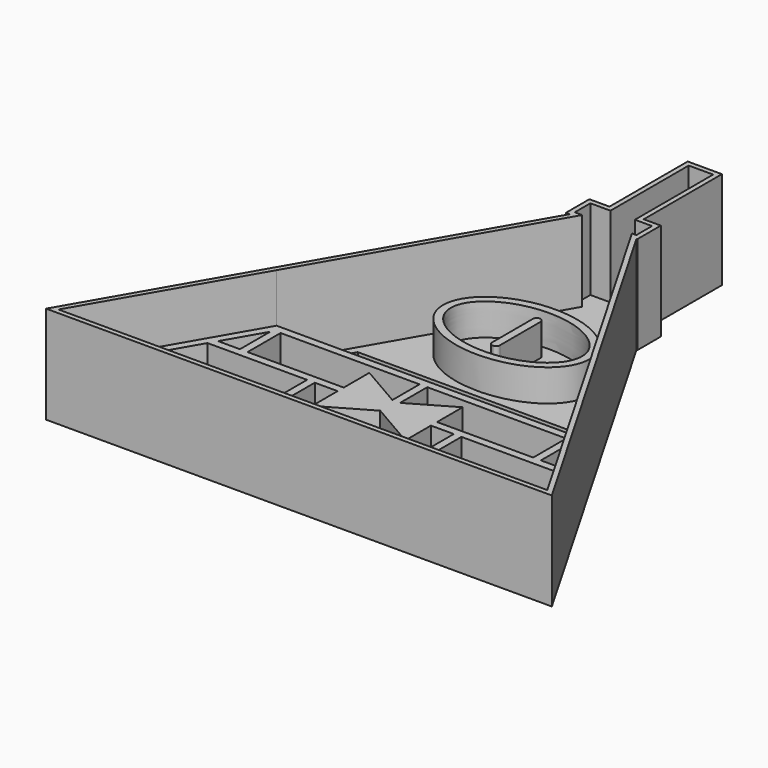
from build123d import *

# Parameters (mm, degrees)
F0_W     = 18.05
F0_H     = 5.358
F1_DEPTH = 6.35
F2_DEPTH = 12.7
F3_DEPTH = 2.2098


# Not quite as in the source:
# - the dataset's text gives a spline's control points without its knots; the knots are read off the source's solid


with BuildPart() as f1:
    # F0 (on Top) → F1 (new body)
    with BuildSketch(Plane.XY):
        Polygon((-73.402151112, 4.5771139196), (-78.1832148198, 4.5771139196), (-82.1426829659, -2.2808860804), (-73.402151112, -2.2808860804), (-63.877151112, -2.2808860804), (-63.877151112, 4.5771139196), align=None)
        Polygon((-64.377151112, -1.7808860804), (-80.6993072929, -1.7808860804), (-77.317189416, 4.0771139196), (-64.377151112, 4.0771139196), align=None, mode=Mode.SUBTRACT)
        Polygon((-73.402151112, -2.2808860804), (-82.1426829659, -2.2808860804), (-86.102151112, -9.1388860804), (-73.402151112, -9.1388860804), align=None)
        Polygon((-84.3701003044, -8.1388860804), (-81.2766575621, -2.7808860804), (-73.902151112, -2.7808860804), (-73.902151112, -8.1388860804), align=None, mode=Mode.SUBTRACT)
        Polygon((-63.877151112, -2.2808860804), (-73.402151112, -2.2808860804), (-73.402151112, -9.1388860804), (-54.352151112, -9.1388860804), (-54.352151112, -2.2808860804), align=None)
        with Locations((-63.877151112, -5.4598860804)):
            Rectangle(F0_W, F0_H, mode=Mode.SUBTRACT)
        Polygon((-73.0690461353, 11.4351139196), (-73.402151112, 11.4351139196), (-73.402151112, 4.5771139196), (-63.877151112, 4.5771139196), (-63.877151112, -2.2808860804), (-54.352151112, -2.2808860804), (-44.827151112, -2.2808860804), (-35.302151112, -2.2808860804), (-26.5616192581, -2.2808860804), (-34.4805555503, 11.4351139196), (-35.302151112, 11.4351139196), (-35.5480732541, 11.4351139196), align=None)
        Polygon((-60.4114715209, 9.2301647272), (-60.4114715209, 5.0771139196), (-72.902151112, 5.0771139196), (-72.902151112, 10.4351139196), (-54.852151112, 10.4351139196), (-54.852151112, 6.0204895926), align=None, mode=Mode.SUBTRACT)
        Polygon((-48.2928307031, -0.0759368879), (-48.2928307031, 4.0771139196), (-45.327151112, 4.0771139196), (-45.327151112, -1.7808860804), (-63.377151112, -1.7808860804), (-63.377151112, 4.0771139196), (-60.4114715209, 4.0771139196), (-60.4114715209, -0.0759368879), (-54.352151112, 3.4224133812), align=None, mode=Mode.SUBTRACT)
        Polygon((-31.387112808, 4.0771139196), (-28.0049949311, -1.7808860804), (-44.327151112, -1.7808860804), (-44.327151112, 4.0771139196), align=None, mode=Mode.SUBTRACT)
        Polygon((-35.802151112, 5.0771139196), (-48.2928307031, 5.0771139196), (-48.2928307031, 9.2301647272), (-53.852151112, 6.0204895926), (-53.852151112, 10.4351139196), (-35.802151112, 10.4351139196), align=None, mode=Mode.SUBTRACT)
        Polygon((-34.802151112, 10.1431388709), (-31.8772802426, 5.0771139196), (-34.802151112, 5.0771139196), align=None, mode=Mode.SUBTRACT)
        Polygon((-73.402151112, 11.4351139196), (-74.2237466737, 11.4351139196), (-78.1832148198, 4.5771139196), (-73.402151112, 4.5771139196), align=None)
        Polygon((-73.902151112, 5.0771139196), (-76.7398391468, 5.0771139196), (-73.902151112, 9.992133772), align=None, mode=Mode.SUBTRACT)
        Polygon((-35.302151112, -2.2808860804), (-35.302151112, -9.1388860804), (-22.602151112, -9.1388860804), (-26.5616192581, -2.2808860804), align=None)
        Polygon((-34.802151112, -2.7808860804), (-27.4276446619, -2.7808860804), (-24.3342019195, -8.1388860804), (-34.802151112, -8.1388860804), align=None, mode=Mode.SUBTRACT)
        Polygon((-54.352151112, -2.2808860804), (-54.352151112, -9.1388860804), (-35.302151112, -9.1388860804), (-35.302151112, -2.2808860804), (-44.827151112, -2.2808860804), align=None)
        with Locations((-44.827151112, -5.4598860804)):
            Rectangle(F0_W, F0_H, mode=Mode.SUBTRACT)
    extrude(amount=F1_DEPTH)

    # F0 (on Top) → F2 (join)
    with BuildSketch(Plane.XY):
        Polygon((-56.5746523037, 56.1289191246), (-56.5746523037, 43.4289191246), (-59.1838299711, 43.4289191246), (-59.1838299711, 39.6189167411), (-58.6850567459, 39.6189167411), (-87.202005439, -9.7738872722), (-21.502296785, -9.7738872722), (-50.019245478, 39.6189167411), (-49.9071499202, 39.6189167411), (-49.9071499202, 43.4289191246), (-52.1296499202, 43.4289191246), (-52.1296499202, 56.1289191246), align=None)
        Polygon((-74.2237466737, 11.4351139196), (-57.5852024189, 40.2539179328), (-58.5488287793, 40.2539179328), (-58.5488287793, 42.7939179328), (-55.939651112, 42.7939179328), (-55.939651112, 55.4939179328), (-52.764651112, 55.4939179328), (-52.764651112, 42.7939179328), (-50.542151112, 42.7939179328), (-50.542151112, 40.2539179328), (-51.119099805, 40.2539179328), (-34.4805555503, 11.4351139196), (-26.5616192581, -2.2808860804), (-22.602151112, -9.1388860804), (-35.302151112, -9.1388860804), (-54.352151112, -9.1388860804), (-73.402151112, -9.1388860804), (-86.102151112, -9.1388860804), (-82.1426829659, -2.2808860804), (-78.1832148198, 4.5771139196), align=None, mode=Mode.SUBTRACT)
    extrude(amount=F2_DEPTH)



with BuildPart() as f1b:
    # F0 (on Top) → F1, piece 2 (new body)
    with BuildSketch(Plane.XY):
        with BuildLine():
            add(Edge.make_bspline(
                [(-54.352145642, 19.1837270599), (-37.8543616999, 19.1837270599), (-46.103253671, 28.7087270599), (-54.352145642, 38.2337270599), (-62.6010376131, 28.7087270599), (-70.8499295841, 19.1837270599), (-54.352145642, 19.1837270599)],
                knots=[4.7123889804, 4.7123889804, 4.7123889804, 6.8067840828, 6.8067840828, 8.9011791852, 8.9011791852, 10.9955742876, 10.9955742876, 10.9955742876], degree=2, weights=[1, 0.5, 1, 0.5, 1, 0.5, 1]))
        make_face()
        with BuildLine():
            add(Edge.make_bspline(
                [(-45.827145642, 25.5337270599), (-45.827145642, 25.8519377152), (-45.9208714076, 26.4883590256), (-46.3482817791, 27.4376066909), (-47.0906705746, 28.3694216685), (-48.1278583866, 29.2134440557), (-49.4278608435, 29.9276027455), (-50.9536840842, 30.4720106822), (-52.334286038, 30.7509003907), (-53.4791973585, 30.8645462988), (-54.352145642, 30.8933174405), (-55.2250939256, 30.8645462988), (-56.3700052461, 30.7509003907), (-57.7506071999, 30.4720106822), (-59.2764304406, 29.9276027455), (-60.5764328975, 29.2134440557), (-61.6136207095, 28.3694216685), (-62.3560095049, 27.4376066909), (-62.7834198764, 26.4883590256), (-62.9240085248, 25.5337270599), (-62.7834198764, 24.5790950943), (-62.3560095049, 23.6298474289), (-61.6136207095, 22.6980324514), (-60.5764328975, 21.8540100641), (-59.2764304406, 21.1398513743), (-57.7506071999, 20.5954434377), (-56.3700052461, 20.3165537291), (-55.2250939256, 20.2029078211), (-54.352145642, 20.1741366794), (-53.4791973585, 20.2029078211), (-52.334286038, 20.3165537291), (-50.9536840842, 20.5954434377), (-49.4278608435, 21.1398513743), (-48.1278583866, 21.8540100641), (-47.0906705746, 22.6980324514), (-46.3482817791, 23.6298474289), (-45.9208714076, 24.5790950943), (-45.827145642, 25.2155164047), (-45.827145642, 25.5337270599)],
                knots=[0, 0, 0, 0, 0.03125, 0.0625, 0.09375, 0.125, 0.15625, 0.1875, 0.21875, 0.234375, 0.25, 0.265625, 0.28125, 0.3125, 0.34375, 0.375, 0.40625, 0.4375, 0.46875, 0.5, 0.53125, 0.5625, 0.59375, 0.625, 0.65625, 0.6875, 0.71875, 0.734375, 0.75, 0.765625, 0.78125, 0.8125, 0.84375, 0.875, 0.90625, 0.9375, 0.96875, 1, 1, 1, 1], degree=3))
        make_face(mode=Mode.SUBTRACT)
    extrude(amount=F1_DEPTH)


with BuildPart() as f1c:
    # F0 (on Top) → F1, piece 3 (new body)
    with BuildSketch(Plane.XY):
        with BuildLine():
            ThreePointArc((-54.352145642, 29.3437270599), (-54.7113558869, 29.1949373048), (-54.860145642, 28.8357270599))
            Line((-54.860145642, 28.8357270599), (-54.860145642, 22.2317270599))
            ThreePointArc((-54.860145642, 22.2317270599), (-54.7113558869, 21.8725168151), (-54.352145642, 21.7237270599))
            ThreePointArc((-54.352145642, 21.7237270599), (-53.9929353972, 21.8725168151), (-53.844145642, 22.2317270599))
            Line((-53.844145642, 22.2317270599), (-53.844145642, 28.8357270599))
            ThreePointArc((-53.844145642, 28.8357270599), (-53.9929353972, 29.1949373048), (-54.352145642, 29.3437270599))
        make_face()
    extrude(amount=F1_DEPTH)


with BuildPart() as f1_1:
    add(f1.part)

    add(f1b.part)  # F3 merges F1b

    add(f1c.part)  # F3 merges F1c
    # F0 (on Top) → F3 (join)
    with BuildSketch(Plane.XY):
        Polygon((-58.5488287793, 40.2539179328), (-57.5852024189, 40.2539179328), (-74.2237466737, 11.4351139196), (-73.402151112, 11.4351139196), (-73.0690461353, 11.4351139196), (-69.1309787943, 18.2560466379), (-39.4861405951, 18.2560466379), (-35.5480732541, 11.4351139196), (-35.302151112, 11.4351139196), (-34.4805555503, 11.4351139196), (-51.119099805, 40.2539179328), (-50.542151112, 40.2539179328), (-50.542151112, 42.7939179328), (-52.764651112, 42.7939179328), (-52.764651112, 55.4939179328), (-55.939651112, 55.4939179328), (-55.939651112, 42.7939179328), (-58.5488287793, 42.7939179328), align=None)
        with BuildLine():
            add(Edge.make_bspline(
                [(-54.352145642, 19.1837270599), (-37.8543616999, 19.1837270599), (-46.103253671, 28.7087270599), (-54.352145642, 38.2337270599), (-62.6010376131, 28.7087270599), (-70.8499295841, 19.1837270599), (-54.352145642, 19.1837270599)],
                knots=[4.7123889804, 4.7123889804, 4.7123889804, 6.8067840828, 6.8067840828, 8.9011791852, 8.9011791852, 10.9955742876, 10.9955742876, 10.9955742876], degree=2, weights=[1, 0.5, 1, 0.5, 1, 0.5, 1]))
        make_face(mode=Mode.SUBTRACT)
        with BuildLine():
            add(Edge.make_bspline(
                [(-54.352145642, 19.1837270599), (-37.8543616999, 19.1837270599), (-46.103253671, 28.7087270599), (-54.352145642, 38.2337270599), (-62.6010376131, 28.7087270599), (-70.8499295841, 19.1837270599), (-54.352145642, 19.1837270599)],
                knots=[4.7123889804, 4.7123889804, 4.7123889804, 6.8067840828, 6.8067840828, 8.9011791852, 8.9011791852, 10.9955742876, 10.9955742876, 10.9955742876], degree=2, weights=[1, 0.5, 1, 0.5, 1, 0.5, 1]))
        make_face()
        with BuildLine():
            add(Edge.make_bspline(
                [(-45.827145642, 25.5337270599), (-45.827145642, 25.8519377152), (-45.9208714076, 26.4883590256), (-46.3482817791, 27.4376066909), (-47.0906705746, 28.3694216685), (-48.1278583866, 29.2134440557), (-49.4278608435, 29.9276027455), (-50.9536840842, 30.4720106822), (-52.334286038, 30.7509003907), (-53.4791973585, 30.8645462988), (-54.352145642, 30.8933174405), (-55.2250939256, 30.8645462988), (-56.3700052461, 30.7509003907), (-57.7506071999, 30.4720106822), (-59.2764304406, 29.9276027455), (-60.5764328975, 29.2134440557), (-61.6136207095, 28.3694216685), (-62.3560095049, 27.4376066909), (-62.7834198764, 26.4883590256), (-62.9240085248, 25.5337270599), (-62.7834198764, 24.5790950943), (-62.3560095049, 23.6298474289), (-61.6136207095, 22.6980324514), (-60.5764328975, 21.8540100641), (-59.2764304406, 21.1398513743), (-57.7506071999, 20.5954434377), (-56.3700052461, 20.3165537291), (-55.2250939256, 20.2029078211), (-54.352145642, 20.1741366794), (-53.4791973585, 20.2029078211), (-52.334286038, 20.3165537291), (-50.9536840842, 20.5954434377), (-49.4278608435, 21.1398513743), (-48.1278583866, 21.8540100641), (-47.0906705746, 22.6980324514), (-46.3482817791, 23.6298474289), (-45.9208714076, 24.5790950943), (-45.827145642, 25.2155164047), (-45.827145642, 25.5337270599)],
                knots=[0, 0, 0, 0, 0.03125, 0.0625, 0.09375, 0.125, 0.15625, 0.1875, 0.21875, 0.234375, 0.25, 0.265625, 0.28125, 0.3125, 0.34375, 0.375, 0.40625, 0.4375, 0.46875, 0.5, 0.53125, 0.5625, 0.59375, 0.625, 0.65625, 0.6875, 0.71875, 0.734375, 0.75, 0.765625, 0.78125, 0.8125, 0.84375, 0.875, 0.90625, 0.9375, 0.96875, 1, 1, 1, 1], degree=3))
        make_face(mode=Mode.SUBTRACT)
        with BuildLine():
            add(Edge.make_bspline(
                [(-45.827145642, 25.5337270599), (-45.827145642, 25.8519377152), (-45.9208714076, 26.4883590256), (-46.3482817791, 27.4376066909), (-47.0906705746, 28.3694216685), (-48.1278583866, 29.2134440557), (-49.4278608435, 29.9276027455), (-50.9536840842, 30.4720106822), (-52.334286038, 30.7509003907), (-53.4791973585, 30.8645462988), (-54.352145642, 30.8933174405), (-55.2250939256, 30.8645462988), (-56.3700052461, 30.7509003907), (-57.7506071999, 30.4720106822), (-59.2764304406, 29.9276027455), (-60.5764328975, 29.2134440557), (-61.6136207095, 28.3694216685), (-62.3560095049, 27.4376066909), (-62.7834198764, 26.4883590256), (-62.9240085248, 25.5337270599), (-62.7834198764, 24.5790950943), (-62.3560095049, 23.6298474289), (-61.6136207095, 22.6980324514), (-60.5764328975, 21.8540100641), (-59.2764304406, 21.1398513743), (-57.7506071999, 20.5954434377), (-56.3700052461, 20.3165537291), (-55.2250939256, 20.2029078211), (-54.352145642, 20.1741366794), (-53.4791973585, 20.2029078211), (-52.334286038, 20.3165537291), (-50.9536840842, 20.5954434377), (-49.4278608435, 21.1398513743), (-48.1278583866, 21.8540100641), (-47.0906705746, 22.6980324514), (-46.3482817791, 23.6298474289), (-45.9208714076, 24.5790950943), (-45.827145642, 25.2155164047), (-45.827145642, 25.5337270599)],
                knots=[0, 0, 0, 0, 0.03125, 0.0625, 0.09375, 0.125, 0.15625, 0.1875, 0.21875, 0.234375, 0.25, 0.265625, 0.28125, 0.3125, 0.34375, 0.375, 0.40625, 0.4375, 0.46875, 0.5, 0.53125, 0.5625, 0.59375, 0.625, 0.65625, 0.6875, 0.71875, 0.734375, 0.75, 0.765625, 0.78125, 0.8125, 0.84375, 0.875, 0.90625, 0.9375, 0.96875, 1, 1, 1, 1], degree=3))
        make_face()
        with BuildLine():
            Line((-54.860145642, 22.2317270599), (-54.860145642, 28.8357270599))
            ThreePointArc((-54.860145642, 28.8357270599), (-54.7113558869, 29.1949373048), (-54.352145642, 29.3437270599))
            ThreePointArc((-54.352145642, 29.3437270599), (-53.9929353972, 29.1949373048), (-53.844145642, 28.8357270599))
            Line((-53.844145642, 28.8357270599), (-53.844145642, 22.2317270599))
            ThreePointArc((-53.844145642, 22.2317270599), (-53.9929353972, 21.8725168151), (-54.352145642, 21.7237270599))
            ThreePointArc((-54.352145642, 21.7237270599), (-54.7113558869, 21.8725168151), (-54.860145642, 22.2317270599))
        make_face(mode=Mode.SUBTRACT)
        with BuildLine():
            ThreePointArc((-54.352145642, 29.3437270599), (-54.7113558869, 29.1949373048), (-54.860145642, 28.8357270599))
            Line((-54.860145642, 28.8357270599), (-54.860145642, 22.2317270599))
            ThreePointArc((-54.860145642, 22.2317270599), (-54.7113558869, 21.8725168151), (-54.352145642, 21.7237270599))
            ThreePointArc((-54.352145642, 21.7237270599), (-53.9929353972, 21.8725168151), (-53.844145642, 22.2317270599))
            Line((-53.844145642, 22.2317270599), (-53.844145642, 28.8357270599))
            ThreePointArc((-53.844145642, 28.8357270599), (-53.9929353972, 29.1949373048), (-54.352145642, 29.3437270599))
        make_face()
    extrude(amount=F3_DEPTH)


solid = f1_1.part
